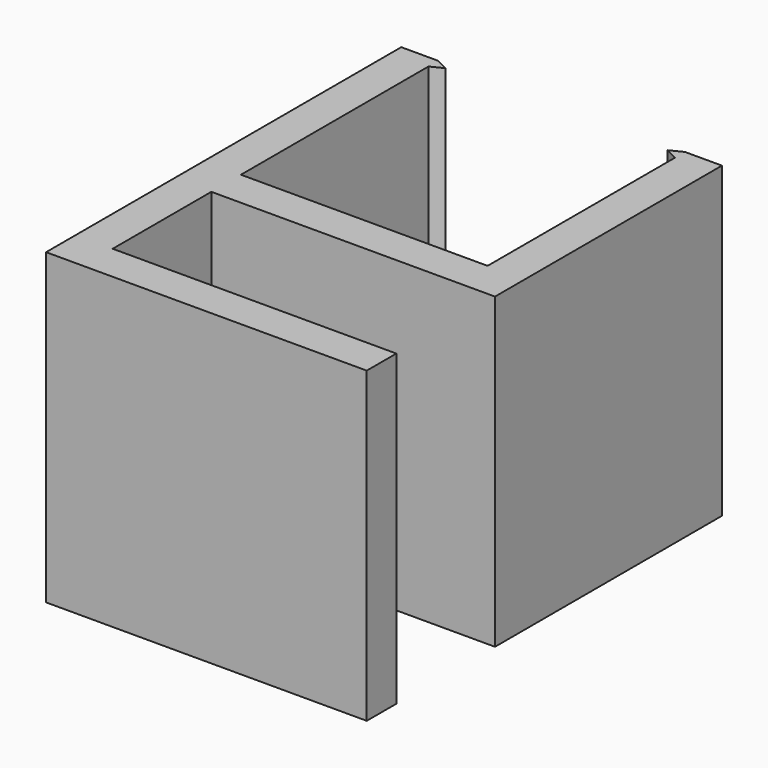
from build123d import *

# Parameters (mm, degrees)
F0_W       = 1
F0_H       = 1
F0_W_2     = 20
F0_H_2     = 3
F0_W_3     = 3
F0_H_3     = 10
F1_DEPTH   = 25
F2_SIZE2   = 0.49999
F2_SIZE    = 0.99999
F2_2_SIZE2 = 0.5
F2_2_SIZE  = 1
F3_SIZE2   = 1
F3_SIZE    = 0.5
F3_2_SIZE2 = 0.99999
F3_2_SIZE  = 0.49999


# Not quite as in the source:
# - a fillet or chamfer is up to 0.001 mm smaller than in the source, because OpenCascade refuses the exact size


with BuildPart() as f1:
    # F0 (on Top) → F1 (new body)
    with BuildSketch(Plane.XY):
        Polygon((-12.6065595312, 12.1843403429), (-15.6065595312, 12.1843403429), (-15.6065595312, -10.8156596571), (-12.6065595312, -10.8156596571), (-12.6065595312, -7.8156596571), (-12.6065595312, 11.1843403429), align=None)
        with Locations((-12.1065595312, 11.6843403429)):
            Rectangle(F0_W, F0_H)
        with Locations((-2.6065595312, -9.3156596571)):
            Rectangle(F0_W_2, F0_H_2)
        Polygon((7.3934404688, -7.8156596571), (7.3934404688, -10.8156596571), (10.3934404688, -10.8156596571), (10.3934404688, 12.1843403429), (7.3934404688, 12.1843403429), (7.3934404688, 11.1843403429), align=None)
        with Locations((-14.1065595312, -15.8156596571)):
            Rectangle(F0_W_3, F0_H_3)
        Polygon((-12.6065595312, -20.8156596571), (-15.6065595312, -20.8156596571), (-15.6065595312, -23.8156596571), (10.3934404688, -23.8156596571), (10.3934404688, -20.8156596571), align=None)
        with Locations((6.8934404688, 11.6843403429)):
            Rectangle(F0_W, F0_H)
    extrude(amount=F1_DEPTH)

    # F2 (size 1 and 0.5 in the source; OpenCascade refuses exactly that, so slightly less here)
    f2_edges = [f1.edges().sort_by_distance(p)[0] for p in [
        (6.39344, 11.18434, 12.5),
    ]]
    f2_side = f1.faces().sort_by_distance((6.89344, 11.18434, 12.5))[0]
    chamfer(f2_edges, length=F2_SIZE, length2=F2_SIZE2, reference=f2_side)

    # F2#2
    f2_2_edges = [f1.edges().sort_by_distance(p)[0] for p in [
        (-11.60656, 12.18434, 12.5),
    ]]
    f2_2_side = f1.faces().sort_by_distance((-13.60656, 12.18434, 12.5))[0]
    chamfer(f2_2_edges, length=F2_2_SIZE, length2=F2_2_SIZE2, reference=f2_2_side)

    # F3
    f3_edges = [f1.edges().sort_by_distance(p)[0] for p in [
        (6.39344, 12.18434, 12.5),
    ]]
    f3_side = f1.faces().sort_by_distance((6.39344, 11.934335, 12.5))[0]
    chamfer(f3_edges, length=F3_SIZE, length2=F3_SIZE2, reference=f3_side)

    # F3#2 (size 0.5 and 1 in the source; OpenCascade refuses exactly that, so slightly less here)
    f3_2_edges = [f1.edges().sort_by_distance(p)[0] for p in [
        (-11.60656, 11.18434, 12.5),
    ]]
    f3_2_side = f1.faces().sort_by_distance((-11.60656, 11.43434, 12.5))[0]
    chamfer(f3_2_edges, length=F3_2_SIZE, length2=F3_2_SIZE2, reference=f3_2_side)


solid = f1.part
